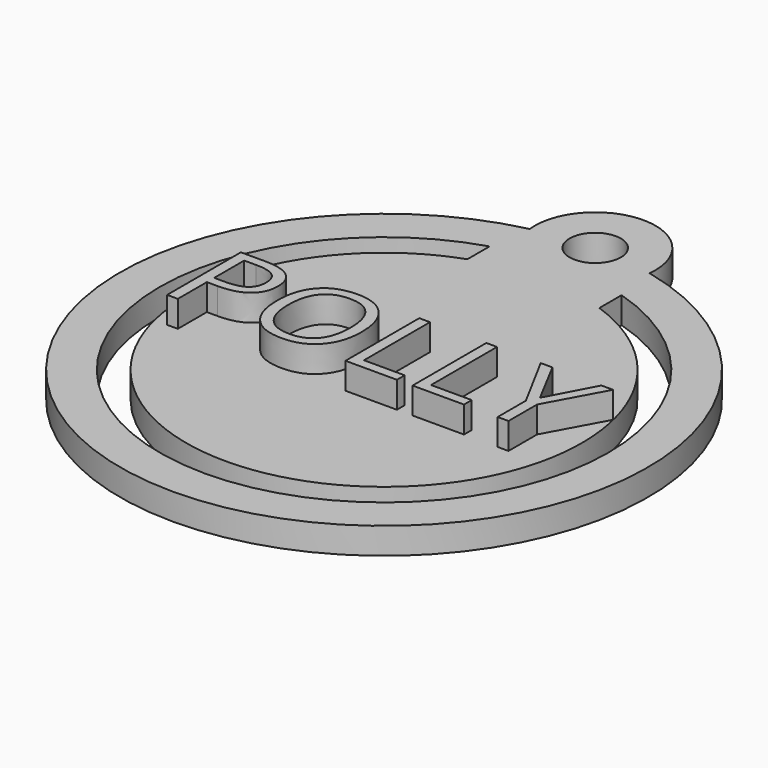
from build123d import *

# Parameters (mm, degrees)
F0_R         = 12.7
F1_DEPTH     = 1.27
F4_DEPTH     = 6.23232
F5_TEXT_SIZE = 6.2159771292
F6_DEPTH     = 1.27
F8_DEPTH     = 1.27
F9_R         = 1.2325218331
F10_DEPTH    = 1.271


# Not quite as in the source:
# - Text() gives the source's letters only with a copy of the font that has no kerning and outlines rounded to 1/6400 em; it was checked with that copy


with BuildPart() as f1:
    # F0 (on Top) → F1 (new body)
    with BuildSketch(Plane.XY):
        Circle(F0_R)
    extrude(amount=F1_DEPTH)

    # F2 (on face) → F4 (cut)
    with BuildSketch(Plane.XY.offset(1.27)):
        with BuildLine():
            Line((-3.175, 8.9802561211), (-3.175, 10.3175287739))
            ThreePointArc((-3.175, 10.3175287739), (0, -10.795), (3.175, 10.3175287739))
            Line((3.175, 10.3175287739), (3.175, 8.9802561211))
            ThreePointArc((3.175, 8.9802561211), (0, -9.525), (-3.175, 8.9802561211))
        make_face()
    extrude(amount=-F4_DEPTH, mode=Mode.SUBTRACT)

    # F5 (on face) → F6 (join)
    with BuildSketch(Plane.XY.offset(1.27)):
        with Locations((-9.2584065601, -2.2377517665)):
            Text('POLLY', F5_TEXT_SIZE, font='Open Sans', text_align=(TextAlign.LEFT, TextAlign.BOTTOM))
    extrude(amount=F6_DEPTH)

    # F7 (on face) → F8 (join)
    with BuildSketch(Plane.XY.offset(1.27)):
        with BuildLine():
            ThreePointArc((-2.8822585744, 12.3686129178), (0, 12.7), (2.8822585744, 12.3686129178))
            ThreePointArc((2.8822585744, 12.3686129178), (0, 15.6012466093), (-2.8822585744, 12.3686129178))
        make_face()
        with BuildLine():
            ThreePointArc((12.7, 0), (9.9472278524, 7.8957367011), (2.8822585744, 12.3686129178))
            ThreePointArc((2.8822585744, 12.3686129178), (0, 12.7), (-2.8822585744, 12.3686129178))
            ThreePointArc((-2.8822585744, 12.3686129178), (-7.8957367011, -9.9472278524), (12.7, 0))
        make_face()
        with BuildLine():
            add(Edge.make_bspline(
                [(-7.6102013744, -0.4924219382), (-6.7545332727, -0.4924219382), (-5.8347629069, 0.2330991423), (-5.8347629069, 2.1998731559), (-7.4975367889, 2.1998731559)],
                knots=[0, 0, 0, 1, 2, 3.9178674352, 3.9178674352, 3.9178674352], degree=2))
            Line((-7.6102013744, -0.4924219382), (-8.1327319518, -0.4924219382))
            Line((-8.1327319518, -0.4924219382), (-8.1327319518, -2.2377517665))
            Line((-8.1327319518, -2.2377517665), (-8.6484638043, -2.2377517665))
            Line((-8.6484638043, -2.2377517665), (-8.6484638043, 2.1998731559))
            Line((-8.6484638043, 2.1998731559), (-7.4975367889, 2.1998731559))
        make_face(mode=Mode.SUBTRACT)
        with BuildLine():
            add(Edge.make_bspline(
                [(-1.0542879959, -0.0126262035), (-1.0542879959, 1.0557448655), (-2.1284865435, 2.2698028986), (-4.0680656572, 2.2698028986), (-5.1364367262, 1.0771122869), (-5.1364367262, -1.0994509547), (-4.0709793964, -2.2989402914), (-2.1323715293, -2.2989402914), (-1.0542879959, -1.0780835334), (-1.0542879959, -0.0126262035)],
                knots=[0, 0, 0, 1, 2, 3.0274111675, 4.054822335, 5.0905190765, 6.1262158179, 7.1393304699, 8.1524451218, 8.1524451218, 8.1524451218], degree=2))
        make_face(mode=Mode.SUBTRACT)
        with BuildLine():
            ThreePointArc((-3.175, 8.9802561211), (0, -9.525), (3.175, 8.9802561211))
            Line((3.175, 8.9802561211), (3.175, 10.3175287739))
            ThreePointArc((3.175, 10.3175287739), (0, -10.795), (-3.175, 10.3175287739))
            Line((-3.175, 10.3175287739), (-3.175, 8.9802561211))
        make_face(mode=Mode.SUBTRACT)
        Polygon((2.4082055144, -2.2377517665), (-0.0655591338, -2.2377517665), (-0.0655591338, 2.1998731559), (0.4501727187, 2.1998731559), (0.4501727187, -1.7705822354), (2.4082055144, -1.7705822354), align=None, mode=Mode.SUBTRACT)
        Polygon((5.634686143, -2.2377517665), (3.1609214949, -2.2377517665), (3.1609214949, 2.1998731559), (3.6766533473, 2.1998731559), (3.6766533473, -1.7705822354), (5.634686143, -1.7705822354), align=None, mode=Mode.SUBTRACT)
        Polygon((6.3417535415, 2.1998731559), (7.5169617175, -0.0194249285), (8.6999398649, 2.1998731559), (9.2584065601, 2.1998731559), (7.7772557597, -0.5167030989), (7.7772557597, -2.2377517665), (7.2556964287, -2.2377517665), (7.2556964287, -0.5409842595), (5.7774593677, 2.1998731559), align=None, mode=Mode.SUBTRACT)
    extrude(amount=-F8_DEPTH)

    # F9 (on face) → F10 (cut, through all)
    with BuildSketch(Plane.XY.offset(1.27)):
        with Locations((0, 12.7)):
            Circle(F9_R)
    extrude(amount=-F10_DEPTH, mode=Mode.SUBTRACT)


solid = f1.part
